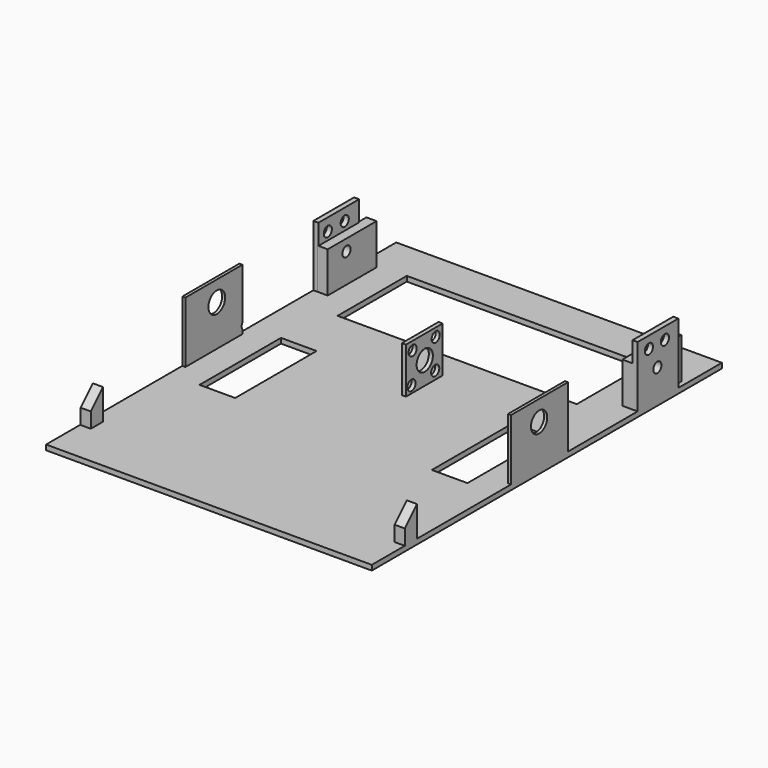
from build123d import *

# Parameters (mm, degrees)
F0_W      = 320
F0_H      = 430
F1_DEPTH  = 5
F2_W      = 35
F2_H      = 100
F3_DEPTH  = 5
F4_W      = 35
F4_H      = 100
F5_DEPTH  = 5
F7_DEPTH  = 5
F8_W      = 3
F8_H      = 70
F9_DEPTH  = 60
F10_W     = 3
F10_H     = 70
F11_DEPTH = 60
F12_W     = 5
F12_H     = 50
F13_DEPTH = 60
F14_W     = 5
F14_H     = 50
F15_DEPTH = 60
F16_R     = 10
F17_DEPTH = 120
F18_R     = 10.2640382995
F19_DEPTH = 240
F20_W     = 10
F20_H     = 15
F21_DEPTH = 30
F22_SIZE  = 14.99999
F23_W     = 10
F23_H     = 15
F24_DEPTH = 30
F25_SIZE  = 14.99999
F26_W     = 4
F26_H     = 45
F27_DEPTH = 45
F28_W     = 10
F28_H     = 60
F29_DEPTH = 40
F30_W     = 10
F30_H     = 60
F31_DEPTH = 40
F32_R     = 5
F33_DEPTH = 240
F34_R     = 5
F35_DEPTH = 240
F36_R     = 5
F37_DEPTH = 250
F38_R     = 5
F39_DEPTH = 300
F40_R     = 5
F41_DEPTH = 300
F42_R     = 5
F43_DEPTH = 300
F44_R     = 10
F45_DEPTH = 207.2868810425
F46_R     = 5
F47_DEPTH = 207.2868810425
F48_R     = 5
F49_DEPTH = 207.2868810425
F50_R     = 5
F51_DEPTH = 207.2868810425
F52_R     = 5
F53_DEPTH = 207.2868810425


# Not quite as in the source:
# - a fillet or chamfer is up to 0.001 mm smaller than in the source, because OpenCascade refuses the exact size


with BuildPart() as f1:
    # F0 (on Top) → F1 (new body)
    with BuildSketch(Plane.XY):
        with Locations((-47.2858810425, 185.3322760761)):
            Rectangle(F0_W, F0_H)
    extrude(amount=F1_DEPTH)

    # F2 (on face) → F3 (cut)
    with BuildSketch(Plane.XY.offset(5)):
        with Locations((-159.7858810425, 171.3026314974)):
            Rectangle(F2_W, F2_H)
    extrude(amount=-F3_DEPTH, mode=Mode.SUBTRACT)

    # F4 (on face) → F5 (cut)
    with BuildSketch(Plane(origin=(0, 0, 0), x_dir=(1, 0, 0), z_dir=(0, 0, -1))):
        with Locations((67.7159577608, -172.2117364407)):
            Rectangle(F4_W, F4_H)
    extrude(amount=-F5_DEPTH, mode=Mode.SUBTRACT)

    # F6 (on face) → F7 (cut)
    with BuildSketch(Plane.XY.offset(5)):
        Polygon((68.7382593751, 362.0384633541), (-166.2617406249, 362.0384633541), (-166.2617406249, 277.0384633541), (-65.0134384632, 277.0384633541), (-48.7617406249, 277.0384633541), (68.7382593751, 277.0384633541), align=None)
    extrude(amount=-F7_DEPTH, mode=Mode.SUBTRACT)

    # F8 (on face) → F9 (join)
    with BuildSketch(Plane.XY.offset(5)):
        with Locations((-205.7858810425, 172.665733695)):
            Rectangle(F8_W, F8_H)
    extrude(amount=F9_DEPTH)

    # F10 (on face) → F11 (join)
    with BuildSketch(Plane.XY.offset(5)):
        with Locations((111.2141189575, 176.3021534681)):
            Rectangle(F10_W, F10_H)
    extrude(amount=F11_DEPTH)

    # F12 (on face) → F13 (join)
    with BuildSketch(Plane.XY.offset(5)):
        with Locations((-204.7858810425, 323.5781848431)):
            Rectangle(F12_W, F12_H)
    extrude(amount=F13_DEPTH)

    # F14 (on face) → F15 (join)
    with BuildSketch(Plane.XY.offset(5)):
        with Locations((110.2141189575, 321.7600047588)):
            Rectangle(F14_W, F14_H)
    extrude(amount=F15_DEPTH)

    # F16 (on Right) → F17 (cut)
    with BuildSketch(Plane.YZ):
        with Locations((175.784942263, 45.0581042336)):
            Circle(F16_R)
    extrude(amount=F17_DEPTH, mode=Mode.SUBTRACT)

    # F18 (on Right) → F19 (cut)
    with BuildSketch(Plane.YZ):
        with Locations((176.2254685163, 45.2939495444)):
            Circle(F18_R)
    extrude(amount=-F19_DEPTH, mode=Mode.SUBTRACT)

    # F20 (on face) → F21 (join)
    with BuildSketch(Plane.XY.offset(5)):
        with Locations((107.7141189575, 18.3457679302)):
            Rectangle(F20_W, F20_H)
    extrude(amount=F21_DEPTH)

    # F22 (size 15 in the source; OpenCascade refuses exactly that, so slightly less here)
    f22_edges = [f1.edges().sort_by_distance(p)[0] for p in [
        (107.714119, 10.845768, 35),
    ]]
    chamfer(f22_edges, length=F22_SIZE)

    # F23 (on face) → F24 (join)
    with BuildSketch(Plane.XY.offset(5)):
        with Locations((-201.83388412, 19.7091826051)):
            Rectangle(F23_W, F23_H)
    extrude(amount=F24_DEPTH)

    # F25 (size 15 in the source; OpenCascade refuses exactly that, so slightly less here)
    f25_edges = [f1.edges().sort_by_distance(p)[0] for p in [
        (-201.833884, 12.209183, 35),
    ]]
    chamfer(f25_edges, length=F25_SIZE)

    # F26 (on face) → F27 (join)
    with BuildSketch(Plane.XY.offset(5)):
        with Locations((-43.3766950369, 227.4395442009)):
            Rectangle(F26_W, F26_H)
    extrude(amount=F27_DEPTH)

    # F28 (on face) → F29 (join)
    with BuildSketch(Plane.XY.offset(5)):
        with Locations((102.7141189575, 326.7600047588)):
            Rectangle(F28_W, F28_H)
    extrude(amount=F29_DEPTH)

    # F30 (on face) → F31 (join)
    with BuildSketch(Plane.XY.offset(5)):
        with Locations((-198.1973099709, 328.5773980618)):
            Rectangle(F30_W, F30_H)
    extrude(amount=F31_DEPTH)

    # F32 (on Right) → F33 (cut)
    with BuildSketch(Plane.YZ):
        with Locations((310.6648027897, 53.3718466759)):
            Circle(F32_R)
    extrude(amount=F33_DEPTH, mode=Mode.SUBTRACT)

    # F34 (on Right) → F35 (cut)
    with BuildSketch(Plane.YZ):
        with Locations((330.2825987339, 53.3718466759)):
            Circle(F34_R)
    extrude(amount=F35_DEPTH, mode=Mode.SUBTRACT)

    # F36 (on Right) → F37 (cut)
    with BuildSketch(Plane.YZ):
        with Locations((321.0507035255, 33.1770926714)):
            Circle(F36_R)
    extrude(amount=F37_DEPTH, mode=Mode.SUBTRACT)

    # F38 (on Right) → F39 (cut)
    with BuildSketch(Plane.YZ):
        with Locations((310.0878298283, 52.794855088)):
            Circle(F38_R)
    extrude(amount=-F39_DEPTH, mode=Mode.SUBTRACT)

    # F40 (on Right) → F41 (cut)
    with BuildSketch(Plane.YZ):
        with Locations((330.8595716953, 53.3718466759)):
            Circle(F40_R)
    extrude(amount=-F41_DEPTH, mode=Mode.SUBTRACT)

    # F42 (on Right) → F43 (cut)
    with BuildSketch(Plane.YZ):
        with Locations((321.627676487, 33.7540879846)):
            Circle(F42_R)
    extrude(amount=-F43_DEPTH, mode=Mode.SUBTRACT)

    # F44 (on Right) → F45 (cut, through all)
    with BuildSketch(Plane.YZ):
        with Locations((228.0015647411, 27.0902961493)):
            Circle(F44_R)
    extrude(amount=-F45_DEPTH, mode=Mode.SUBTRACT)

    # F46 (on Right) → F47 (cut, through all)
    with BuildSketch(Plane.YZ):
        with Locations((241.425678134, 41.8319888413)):
            Circle(F46_R)
    extrude(amount=-F47_DEPTH, mode=Mode.SUBTRACT)

    # F48 (on Right) → F49 (cut, through all)
    with BuildSketch(Plane.YZ):
        with Locations((240.8486753702, 12.9823405296)):
            Circle(F48_R)
    extrude(amount=-F49_DEPTH, mode=Mode.SUBTRACT)

    # F50 (on Right) → F51 (cut, through all)
    with BuildSketch(Plane.YZ):
        with Locations((213.0800783634, 41.6209772229)):
            Circle(F50_R)
    extrude(amount=-F51_DEPTH, mode=Mode.SUBTRACT)

    # F52 (on Right) → F53 (cut, through all)
    with BuildSketch(Plane.YZ):
        with Locations((211.7366492748, 12.104251422)):
            Circle(F52_R)
    extrude(amount=-F53_DEPTH, mode=Mode.SUBTRACT)


solid = f1.part
